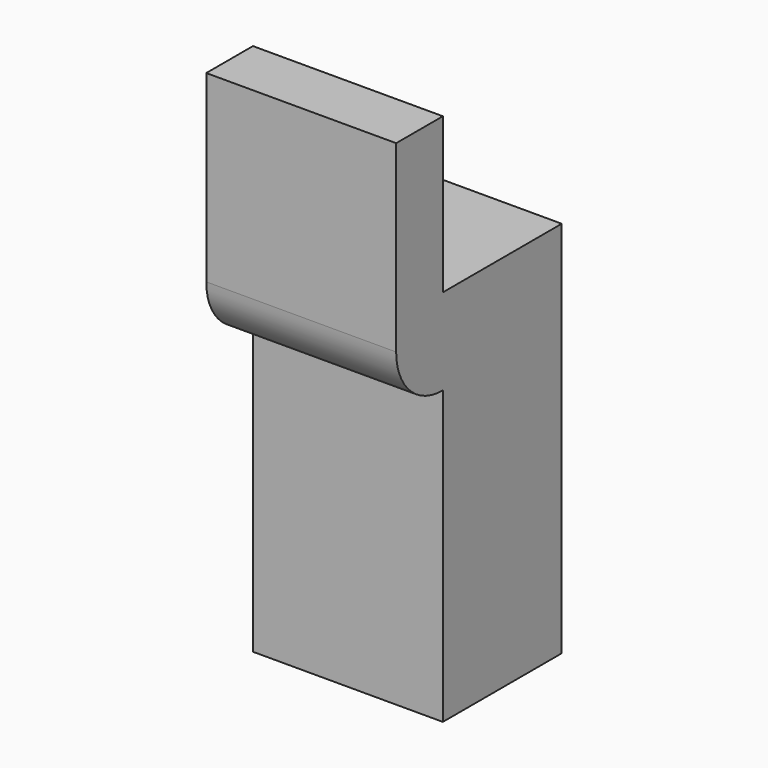
from build123d import *

# Parameters (mm, degrees)
F0_W     = 44.6442011744
F0_H     = 34.9367577583
F1_DEPTH = 88.9
F2_W     = 44.6442011744
F2_H     = 56.7069426179
F3_DEPTH = 13.716
F4_R     = 13.4906253865


with BuildPart() as f1:
    # F0 (on Top) → F1 (new body)
    with BuildSketch(Plane.XY):
        with Locations((33.164284192, 7.5076622888)):
            Rectangle(F0_W, F0_H)
    extrude(amount=F1_DEPTH)

    # F2 (on face) → F3 (join)
    with BuildSketch(Plane.XZ.offset(9.9607165903)):
        with Locations((33.164284192, 96.9944112003)):
            Rectangle(F2_W, F2_H)
    extrude(amount=F3_DEPTH)

    # F4
    f4_edges = [f1.edges().sort_by_distance(p)[0] for p in [
        (33.164284, -23.676717, 68.64094),
    ]]
    fillet(f4_edges, radius=F4_R)


solid = f1.part
